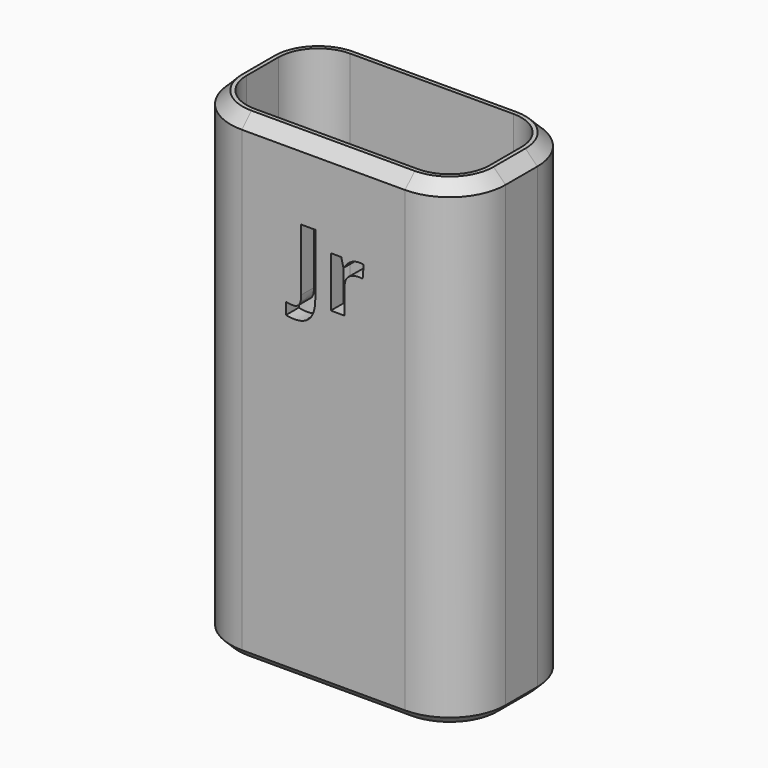
from build123d import *

# Parameters (mm, degrees)
F0_W         = 26.5
F0_H         = 11
F1_DEPTH     = 2
F2_DEPTH     = 60
F3_W         = 7
F3_H         = 4
F4_DEPTH     = 25
F5_TEXT_SIZE = 11.6242864556
F6_DEPTH     = 25
F7_SIZE      = 1
F8_SIZE      = 1.5


# Not quite as in the source:
# - Text() gives the source's letters only with a copy of the font that has no kerning and outlines rounded to 1/6400 em; it was checked with that copy


with BuildPart() as f1:
    # F0 (on Top) → F1 (new body)
    with BuildSketch(Plane.XY):
        with BuildLine():
            Line((25.5, 17), (5, 17))
            ThreePointArc((5, 17), (0.0502525317, 14.9497474683), (-2, 10))
            Line((-2, 10), (-2, 5))
            ThreePointArc((-2, 5), (0.0502525317, 0.0502525317), (5, -2))
            Line((5, -2), (25.5, -2))
            ThreePointArc((25.5, -2), (30.4497474683, 0.0502525317), (32.5, 5))
            Line((32.5, 5), (32.5, 10))
            ThreePointArc((32.5, 10), (30.4497474683, 14.9497474683), (25.5, 17))
        make_face()
        with BuildLine():
            Line((25.5, 0), (5, 0))
            ThreePointArc((5, 0), (1.4644660941, 1.4644660941), (0, 5))
            Line((0, 5), (0, 10))
            ThreePointArc((0, 10), (1.4644660941, 13.5355339059), (5, 15))
            Line((5, 15), (25.5, 15))
            ThreePointArc((25.5, 15), (29.0355339059, 13.5355339059), (30.5, 10))
            Line((30.5, 10), (30.5, 5))
            ThreePointArc((30.5, 5), (29.0355339059, 1.4644660941), (25.5, 0))
        make_face(mode=Mode.SUBTRACT)
        with BuildLine():
            ThreePointArc((0, 5), (1.4644660941, 1.4644660941), (5, 0))
            Line((5, 0), (25.5, 0))
            ThreePointArc((25.5, 0), (29.0355339059, 1.4644660941), (30.5, 5))
            Line((30.5, 5), (30.5, 10))
            ThreePointArc((30.5, 10), (29.0355339059, 13.5355339059), (25.5, 15))
            Line((25.5, 15), (5, 15))
            ThreePointArc((5, 15), (1.4644660941, 13.5355339059), (0, 10))
            Line((0, 10), (0, 5))
        make_face()
        with Locations((15.25, 7.5)):
            Rectangle(F0_W, F0_H, mode=Mode.SUBTRACT)
    extrude(amount=F1_DEPTH)

    # F0 (on Top) → F2 (join)
    with BuildSketch(Plane.XY):
        with BuildLine():
            Line((25.5, 17), (5, 17))
            ThreePointArc((5, 17), (0.0502525317, 14.9497474683), (-2, 10))
            Line((-2, 10), (-2, 5))
            ThreePointArc((-2, 5), (0.0502525317, 0.0502525317), (5, -2))
            Line((5, -2), (25.5, -2))
            ThreePointArc((25.5, -2), (30.4497474683, 0.0502525317), (32.5, 5))
            Line((32.5, 5), (32.5, 10))
            ThreePointArc((32.5, 10), (30.4497474683, 14.9497474683), (25.5, 17))
        make_face()
        with BuildLine():
            Line((25.5, 0), (5, 0))
            ThreePointArc((5, 0), (1.4644660941, 1.4644660941), (0, 5))
            Line((0, 5), (0, 10))
            ThreePointArc((0, 10), (1.4644660941, 13.5355339059), (5, 15))
            Line((5, 15), (25.5, 15))
            ThreePointArc((25.5, 15), (29.0355339059, 13.5355339059), (30.5, 10))
            Line((30.5, 10), (30.5, 5))
            ThreePointArc((30.5, 5), (29.0355339059, 1.4644660941), (25.5, 0))
        make_face(mode=Mode.SUBTRACT)
    extrude(amount=F2_DEPTH)

    # F3 (on Front) → F4 (cut)
    with BuildSketch(Plane.XZ):
        with Locations((16, 27.0405690297)):
            Rectangle(F3_W, F3_H)
    extrude(amount=-F4_DEPTH, mode=Mode.SUBTRACT)

    # F5 (on Front) → F6 (cut)
    with BuildSketch(Plane.XZ):
        with Locations((11.4166227651, 42.1447848945)):
            Text('Jr', F5_TEXT_SIZE, font='Open Sans', font_style=FontStyle.BOLD, text_align=(TextAlign.LEFT, TextAlign.BOTTOM))
    extrude(amount=F6_DEPTH, mode=Mode.SUBTRACT)

    # F7
    f7_edges = [f1.edges().sort_by_distance(p)[0] for p in [
        (15.25, -2, 0),
        (0.050253, 0.050253, 0),
        (-2, 7.5, 0),
        (0.050253, 14.949747, 0),
        (15.25, 17, 0),
        (30.449747, 14.949747, 0),
        (32.5, 7.5, 0),
        (30.449747, 0.050253, 0),
    ]]
    chamfer(f7_edges, length=F7_SIZE)

    # F8
    f8_edges = [f1.edges().sort_by_distance(p)[0] for p in [
        (15.25, -2, 60),
        (30.449747, 0.050253, 60),
        (32.5, 7.5, 60),
        (30.449747, 14.949747, 60),
        (15.25, 17, 60),
        (0.050253, 14.949747, 60),
        (-2, 7.5, 60),
        (0.050253, 0.050253, 60),
    ]]
    chamfer(f8_edges, length=F8_SIZE)


solid = f1.part
